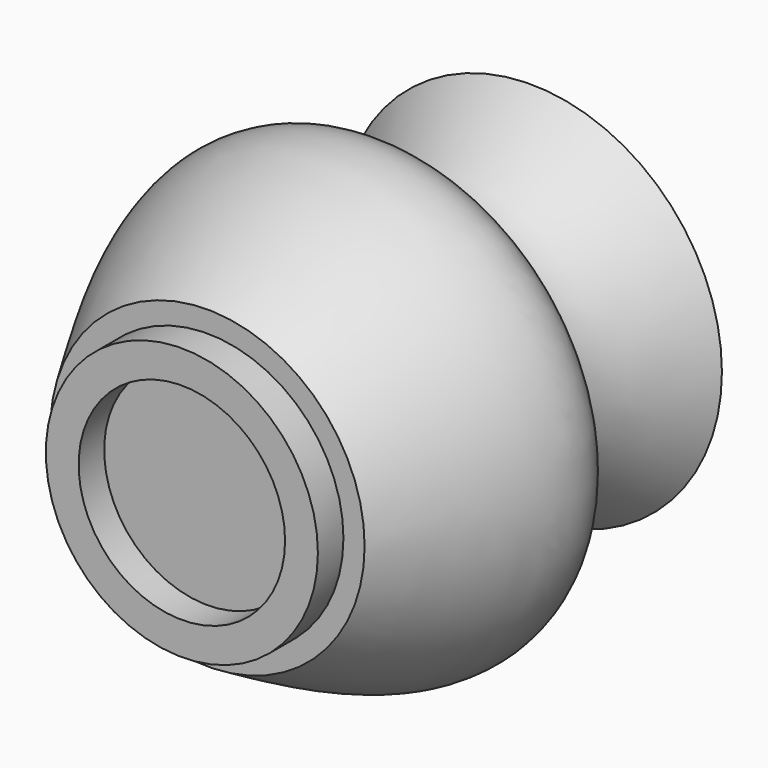
from build123d import *

# Parameters (mm, degrees)
F2_T = 2.5


# Not quite as in the source:
# - a shell that OpenCascade refuses in one call is made with other operations: the cavity is built on its own and cut out


with BuildPart() as f1:
    # F0 (on Top) → F1 (revolve)
    with BuildSketch(Plane.XY):
        with BuildLine():
            Line((38.5857522488, -17.3760261387), (15.9575715661, -17.3760261387))
            Line((15.9575715661, -17.3760261387), (15.9575715661, -65.248735249))
            Line((15.9575715661, -65.248735249), (28.1796697527, -65.248735249))
            Line((28.1796697527, -65.248735249), (28.1796697527, -69.0309181809))
            Line((28.1796697527, -69.0309181809), (32.0662781596, -69.0309181809))
            Line((32.0662781596, -69.0309181809), (32.0662781596, -65.248735249))
            Line((32.0662781596, -65.248735249), (34.5737710595, -65.248735249))
            add(Edge.make_bspline(
                [(38.5857522488, -17.3760261387), (34.1483461344, -23.0657243016), (25.6305257678, -33.9873811535), (49.8326224619, -38.9447863561), (40.1500059988, -55.6361507242), (34.5737710595, -65.248735249)],
                knots=[0, 0, 0, 0, 0.3156320779, 0.6058713744, 1, 1, 1, 1], degree=3))
        make_face()
    revolve(axis=Axis((15.9575715661, -41.3123806939, 0), (0, -1, 0)))

    # F2: shell of thickness 2.5, made by hand


with BuildPart() as f2_core1:
    # F2_t2: copy of F1
    add(f1.part)

    # the walls: a layer under each face that stays
    f2_faces = [f2_core1.faces().sort_by_distance(p)[0] for p in [
        (15.9575715661, -65.248735249, 0),
        (3.7354733795, -67.139826715, 0),
        (26.6967092951, -69.0309181809, -10.739137729),
        (-0.1511350274, -67.139826715, 0),
        (28.3683712284, -65.248735249, -12.4107996623),
        (-6.7644266642, -37.3801254436, 0),
    ]]
    thicken(f2_faces, amount=-F2_T, mode=Mode.SUBTRACT)

    # F2_s3 → F2_t4 (revolve, cut)
    with BuildSketch(Plane.XY):
        Polygon((28.1546697527, -65.273735249), (28.1796697527, -62.748735249), (30.6796697527, -62.748735249), (30.6796697527, -65.248735249), align=None)
    revolve(axis=Axis((15.9575715661, -65.248735249, 0), (0, -1, 0)), mode=Mode.SUBTRACT)

    # F2_s5 → F2_t6 (revolve, cut)
    with BuildSketch(Plane.XY):
        Polygon((32.0912781596, -65.273735249), (29.5662781596, -65.248735249), (29.5662781596, -62.748735249), (32.0662781596, -62.748735249), align=None)
    revolve(axis=Axis((15.9575715661, -65.248735249, 0), (0, -1, 0)), mode=Mode.SUBTRACT)


with BuildPart() as f1_1:
    add(f1.part)

    # what is left inside the walls is the cavity
    f2_cavity = [f2_core1.part.solids().sort_by_distance(p)[0] for p in [
        (1.483034, -35.002243, 0),
    ]]
    add(f2_cavity, mode=Mode.SUBTRACT)


solid = f1_1.part
